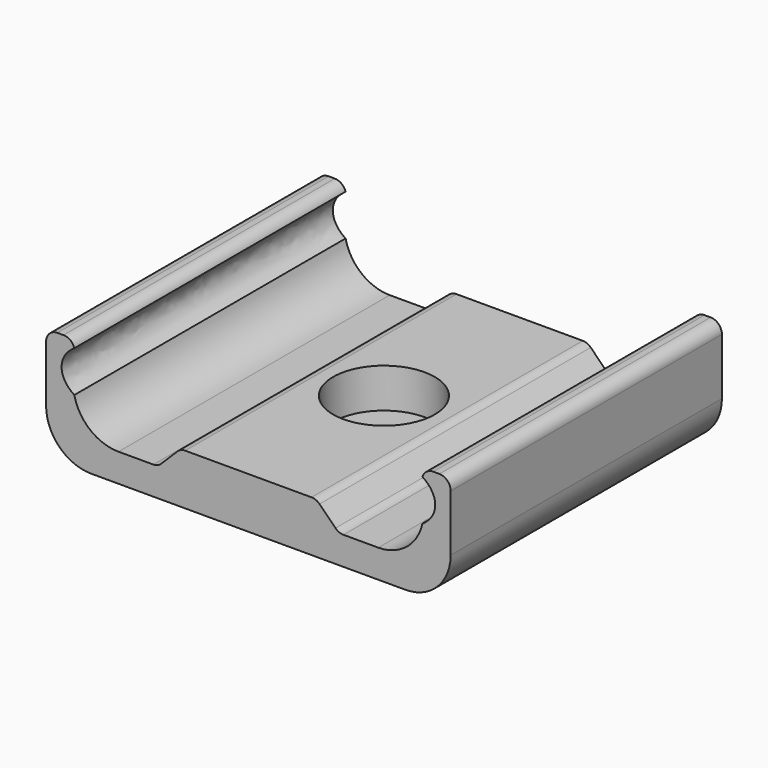
from build123d import *

# Parameters (mm, degrees)
F1_DEPTH       = 30
F3_D           = 4.5
F3_CBORE_D     = 9
F3_CBORE_DEPTH = 3.5
F4_DEPTH       = 30.0010001
F5_T1_DEPTH    = 30
F5_T3_DEPTH    = 30
F5_T5_DEPTH    = 34.788525759
F5_T7_DEPTH    = 35
F5_T9_DEPTH    = 32.0710678119
F5_T11_DEPTH   = 32.0710678119
F5_T13_DEPTH   = 34.7881858635
F5_T15_DEPTH   = 35
F6_T1_DEPTH    = 30
F6_T3_DEPTH    = 30
F6_T5_DEPTH    = 50
F6_T7_DEPTH    = 50


# Not quite as in the source:
# - a fillet or chamfer that OpenCascade refuses, or shapes differently, is made with other operations: its cross-section is extruded or revolved along the edge and cut away or added


with BuildPart() as f1:
    # F0 (on Front) → F1 (new body)
    with BuildSketch(Plane.XZ):
        with BuildLine():
            Line((-17.9, 10), (-17.9, 0))
            Line((-17.9, 0), (17.9, 0))
            Line((17.9, 0), (17.9, 10))
            Line((17.9, 10), (15.4, 10))
            Line((15.4, 10), (15.4, 9.2879775086))
            add(Edge.make_bspline(
                [(15.4, 5.6440113938), (18.1981581314, 7.4659944512), (15.4, 9.2879775086)],
                knots=[2.3143184253, 2.3143184253, 2.3143184253, 3.9688668818, 3.9688668818, 3.9688668818], degree=2, weights=[1, 0.676884683, 1]))
            Line((15.4, 5.6440113938), (15.4, 2.5))
            Line((15.4, 2.5), (8, 2.5))
            Line((8, 2.5), (6, 4.5))
            Line((6, 4.5), (-6, 4.5))
            Line((-6, 4.5), (-8, 2.5))
            Line((-8, 2.5), (-15.4, 2.5))
            Line((-15.4, 2.5), (-15.4, 5.6442375475))
            add(Edge.make_bspline(
                [(-16.5293519812, 7.4659944512), (-16.5293519812, 6.3796188728), (-15.4, 5.6442375475)],
                knots=[0, 0, 0, 0.8272362915, 0.8272362915, 0.8272362915], degree=2, weights=[1, 0.9156725963, 1]))
            add(Edge.make_bspline(
                [(-15.4, 9.2877513548), (-16.5293519812, 8.5523700296), (-16.5293519812, 7.4659944512)],
                knots=[5.4559490157, 5.4559490157, 5.4559490157, 6.2831853072, 6.2831853072, 6.2831853072], degree=2, weights=[1, 0.9156725963, 1]))
            Line((-15.4, 9.2877513548), (-15.4, 10))
            Line((-15.4, 10), (-17.9, 10))
        make_face()
        with BuildLine():
            add(Edge.make_bspline(
                [(-15.4, 5.6442375475), (-9.5383519812, 1.8274058066), (-9.5383519812, 7.4659944512), (-9.5383519812, 13.1045830958), (-15.4, 9.2877513548)],
                knots=[0.8272362915, 0.8272362915, 0.8272362915, 3.1415926536, 3.1415926536, 5.4559490157, 5.4559490157, 5.4559490157], degree=2, weights=[1, 0.4019249885, 1, 0.4019249885, 1]))
            Line((-15.4, 9.2877513548), (-15.4, 5.6442375475))
        make_face()
        with BuildLine():
            Line((-15.4, 5.6442375475), (-15.4, 9.2877513548))
            add(Edge.make_bspline(
                [(-15.4, 9.2877513548), (-16.5293519812, 8.5523700296), (-16.5293519812, 7.4659944512)],
                knots=[5.4559490157, 5.4559490157, 5.4559490157, 6.2831853072, 6.2831853072, 6.2831853072], degree=2, weights=[1, 0.9156725963, 1]))
            add(Edge.make_bspline(
                [(-16.5293519812, 7.4659944512), (-16.5293519812, 6.3796188728), (-15.4, 5.6442375475)],
                knots=[0, 0, 0, 0.8272362915, 0.8272362915, 0.8272362915], degree=2, weights=[1, 0.9156725963, 1]))
        make_face()
        with BuildLine():
            add(Edge.make_bspline(
                [(15.4, 5.6440113938), (18.1981581314, 7.4659944512), (15.4, 9.2879775086)],
                knots=[2.3143184253, 2.3143184253, 2.3143184253, 3.9688668818, 3.9688668818, 3.9688668818], degree=2, weights=[1, 0.676884683, 1]))
            Line((15.4, 9.2879775086), (15.4, 5.6440113938))
        make_face()
        with BuildLine():
            Line((15.4, 5.6440113938), (15.4, 9.2879775086))
            add(Edge.make_bspline(
                [(15.4, 9.2879775086), (9.5382216203, 13.1047957127), (9.5382216203, 7.4659944512)],
                knots=[3.9688668818, 3.9688668818, 3.9688668818, 6.2831853072, 6.2831853072, 6.2831853072], degree=2, weights=[1, 0.4019423572, 1]))
            add(Edge.make_bspline(
                [(9.5382216203, 7.4659944512), (9.5382216203, 1.8271931896), (15.4, 5.6440113938)],
                knots=[0, 0, 0, 2.3143184253, 2.3143184253, 2.3143184253], degree=2, weights=[1, 0.4019423572, 1]))
        make_face()
    extrude(amount=F1_DEPTH)

    # F3 (through all)
    with Locations(Plane.XY.offset(4.5)):
        with Locations((-0.0060852617, -15)):
            CounterBoreHole(F3_D / 2, F3_CBORE_D / 2, F3_CBORE_DEPTH)

    # F0 (on Front) → F4 (cut, through all)
    with BuildSketch(Plane.XZ):
        with BuildLine():
            Line((15.4, 5.6440113938), (15.4, 9.2879775086))
            add(Edge.make_bspline(
                [(15.4, 9.2879775086), (9.5382216203, 13.1047957127), (9.5382216203, 7.4659944512)],
                knots=[3.9688668818, 3.9688668818, 3.9688668818, 6.2831853072, 6.2831853072, 6.2831853072], degree=2, weights=[1, 0.4019423572, 1]))
            add(Edge.make_bspline(
                [(9.5382216203, 7.4659944512), (9.5382216203, 1.8271931896), (15.4, 5.6440113938)],
                knots=[0, 0, 0, 2.3143184253, 2.3143184253, 2.3143184253], degree=2, weights=[1, 0.4019423572, 1]))
        make_face()
        with BuildLine():
            add(Edge.make_bspline(
                [(15.4, 5.6440113938), (18.1981581314, 7.4659944512), (15.4, 9.2879775086)],
                knots=[2.3143184253, 2.3143184253, 2.3143184253, 3.9688668818, 3.9688668818, 3.9688668818], degree=2, weights=[1, 0.676884683, 1]))
            Line((15.4, 9.2879775086), (15.4, 5.6440113938))
        make_face()
        with BuildLine():
            add(Edge.make_bspline(
                [(-15.4, 5.6442375475), (-9.5383519812, 1.8274058066), (-9.5383519812, 7.4659944512), (-9.5383519812, 13.1045830958), (-15.4, 9.2877513548)],
                knots=[0.8272362915, 0.8272362915, 0.8272362915, 3.1415926536, 3.1415926536, 5.4559490157, 5.4559490157, 5.4559490157], degree=2, weights=[1, 0.4019249885, 1, 0.4019249885, 1]))
            Line((-15.4, 9.2877513548), (-15.4, 5.6442375475))
        make_face()
        with BuildLine():
            Line((-15.4, 5.6442375475), (-15.4, 9.2877513548))
            add(Edge.make_bspline(
                [(-15.4, 9.2877513548), (-16.5293519812, 8.5523700296), (-16.5293519812, 7.4659944512)],
                knots=[5.4559490157, 5.4559490157, 5.4559490157, 6.2831853072, 6.2831853072, 6.2831853072], degree=2, weights=[1, 0.9156725963, 1]))
            add(Edge.make_bspline(
                [(-16.5293519812, 7.4659944512), (-16.5293519812, 6.3796188728), (-15.4, 5.6442375475)],
                knots=[0, 0, 0, 0.8272362915, 0.8272362915, 0.8272362915], degree=2, weights=[1, 0.9156725963, 1]))
        make_face()
    extrude(amount=F4_DEPTH, mode=Mode.SUBTRACT)

    # F5: fillet of radius 1 on 8 edges, made by hand

    # F5_s2 → F5_t1 (join)
    with BuildSketch(Plane.XZ):
        with BuildLine():
            ThreePointArc((-8.4142135624, 2.5), (-8.03153013, 2.5761204675), (-7.7071067812, 2.7928932188))
            Line((-7.7071067812, 2.7928932188), (-7.6929646456, 2.7787510832))
            Line((-7.6929646456, 2.7787510832), (-7.9917157288, 2.48))
            Line((-7.9917157288, 2.48), (-8.4142135624, 2.48))
            Line((-8.4142135624, 2.48), (-8.4142135624, 2.5))
        make_face()
    extrude(amount=F5_T1_DEPTH)

    # F5_s4 → F5_t3 (join)
    with BuildSketch(Plane.XZ):
        with BuildLine():
            ThreePointArc((7.7071067812, 2.7928932188), (8.03153013, 2.5761204675), (8.4142135624, 2.5))
            Line((8.4142135624, 2.5), (8.4142135624, 2.48))
            Line((8.4142135624, 2.48), (7.9917157288, 2.48))
            Line((7.9917157288, 2.48), (7.6929646456, 2.7787510832))
            Line((7.6929646456, 2.7787510832), (7.7071067812, 2.7928932188))
        make_face()
    extrude(amount=F5_T3_DEPTH)

    # F5_s6 → F5_t5 (cut)
    with BuildSketch(Plane.XZ.offset(-2.3942628795)):
        with BuildLine():
            ThreePointArc((-15.4, 9.2877513548), (-15.7609436227, 9.8024186422), (-16.3577051518, 10))
            Line((-16.3577051518, 10), (-16.3577051518, 10.02))
            Line((-16.3577051518, 10.02), (-15.4, 10.02))
            Line((-15.4, 10.02), (-15.38, 10))
            ThreePointArc((-15.38, 10), (-15.38, 9.6438756774), (-15.380845897, 9.2935063819))
            Line((-15.380845897, 9.2935063819), (-15.4, 9.2877513548))
        make_face()
    extrude(amount=F5_T5_DEPTH, mode=Mode.SUBTRACT)

    # F5_s8 → F5_t7 (cut)
    with BuildSketch(Plane.XZ.offset(-2.5)):
        with BuildLine():
            ThreePointArc((-17.9, 9), (-17.6071067812, 9.7071067812), (-16.9, 10))
            Line((-16.9, 10), (-16.9, 10.02))
            Line((-16.9, 10.02), (-17.92, 10.02))
            Line((-17.92, 10.02), (-17.92, 9))
            Line((-17.92, 9), (-17.9, 9))
        make_face()
    extrude(amount=F5_T7_DEPTH, mode=Mode.SUBTRACT)

    # F5_s10 → F5_t9 (cut)
    with BuildSketch(Plane.XZ.offset(-1.0355339059)):
        with BuildLine():
            ThreePointArc((-6.2928932188, 4.2071067812), (-5.96846987, 4.4238795325), (-5.5857864376, 4.5))
            Line((-5.5857864376, 4.5), (-5.5857864376, 4.52))
            Line((-5.5857864376, 4.52), (-6.0082842712, 4.52))
            Line((-6.0082842712, 4.52), (-6.3070353544, 4.2212489168))
            Line((-6.3070353544, 4.2212489168), (-6.2928932188, 4.2071067812))
        make_face()
    extrude(amount=F5_T9_DEPTH, mode=Mode.SUBTRACT)

    # F5_s12 → F5_t11 (cut)
    with BuildSketch(Plane.XZ.offset(-1.0355339059)):
        with BuildLine():
            ThreePointArc((5.5857864376, 4.5), (5.96846987, 4.4238795325), (6.2928932188, 4.2071067812))
            Line((6.2928932188, 4.2071067812), (6.3070353544, 4.2212489168))
            Line((6.3070353544, 4.2212489168), (6.0082842712, 4.52))
            Line((6.0082842712, 4.52), (5.5857864376, 4.52))
            Line((5.5857864376, 4.52), (5.5857864376, 4.5))
        make_face()
    extrude(amount=F5_T11_DEPTH, mode=Mode.SUBTRACT)

    # F5_s14 → F5_t13 (cut)
    with BuildSketch(Plane.XZ.offset(-2.3940929318)):
        with BuildLine():
            ThreePointArc((15.4, 9.2879775086), (15.7609703932, 9.8024890992), (16.3576371727, 10))
            Line((16.3576371727, 10), (16.3576371727, 10.02))
            Line((16.3576371727, 10.02), (15.4, 10.02))
            Line((15.4, 10.02), (15.38, 10))
            ThreePointArc((15.38, 10), (15.38, 9.6439887543), (15.3808472565, 9.2937370588))
            Line((15.3808472565, 9.2937370588), (15.4, 9.2879775086))
        make_face()
    extrude(amount=F5_T13_DEPTH, mode=Mode.SUBTRACT)

    # F5_s16 → F5_t15 (cut)
    with BuildSketch(Plane.XZ.offset(-2.5)):
        with BuildLine():
            ThreePointArc((16.9, 10), (17.6071067812, 9.7071067812), (17.9, 9))
            Line((17.9, 9), (17.92, 9))
            Line((17.92, 9), (17.92, 10.02))
            Line((17.92, 10.02), (16.9, 10.02))
            Line((16.9, 10.02), (16.9, 10))
        make_face()
    extrude(amount=F5_T15_DEPTH, mode=Mode.SUBTRACT)

    # F6: fillet of radius 4 on 4 edges, made by hand

    # F6_s2 → F6_t1 (join)
    with BuildSketch(Plane.XZ):
        with BuildLine():
            ThreePointArc((-15.4, 5.6442375475), (-14.000296538, 3.3836680368), (-11.4926133254, 2.5))
            Line((-11.4926133254, 2.5), (-11.4926133254, 2.42))
            Line((-11.4926133254, 2.42), (-15.4, 2.42))
            Line((-15.4, 2.42), (-15.48, 2.5))
            ThreePointArc((-15.48, 2.5), (-15.48, 4.0721187738), (-15.4781477335, 5.6271222985))
            Line((-15.4781477335, 5.6271222985), (-15.4, 5.6442375475))
        make_face()
    extrude(amount=F6_T1_DEPTH)

    # F6_s4 → F6_t3 (join)
    with BuildSketch(Plane.XZ):
        with BuildLine():
            ThreePointArc((11.4926628625, 2.5), (14.0002558892, 3.3835954671), (15.4, 5.6440113938))
            Line((15.4, 5.6440113938), (15.4781467427, 5.6268916217))
            ThreePointArc((15.4781467427, 5.6268916217), (15.48, 4.0720056969), (15.48, 2.5))
            Line((15.48, 2.5), (15.4, 2.42))
            Line((15.4, 2.42), (11.4926628625, 2.42))
            Line((11.4926628625, 2.42), (11.4926628625, 2.5))
        make_face()
    extrude(amount=F6_T3_DEPTH)

    # F6_s6 → F6_t5 (cut)
    with BuildSketch(Plane.XZ.offset(-10)):
        with BuildLine():
            ThreePointArc((17.9, 4), (16.7284271247, 1.1715728753), (13.9, 0))
            Line((13.9, 0), (13.9, -0.08))
            Line((13.9, -0.08), (17.98, -0.08))
            Line((17.98, -0.08), (17.98, 4))
            Line((17.98, 4), (17.9, 4))
        make_face()
    extrude(amount=F6_T5_DEPTH, mode=Mode.SUBTRACT)

    # F6_s8 → F6_t7 (cut)
    with BuildSketch(Plane.XZ.offset(-10)):
        with BuildLine():
            ThreePointArc((-13.9, 0), (-16.7284271247, 1.1715728753), (-17.9, 4))
            Line((-17.9, 4), (-17.98, 4))
            Line((-17.98, 4), (-17.98, -0.08))
            Line((-17.98, -0.08), (-13.9, -0.08))
            Line((-13.9, -0.08), (-13.9, 0))
        make_face()
    extrude(amount=F6_T7_DEPTH, mode=Mode.SUBTRACT)


solid = f1.part
